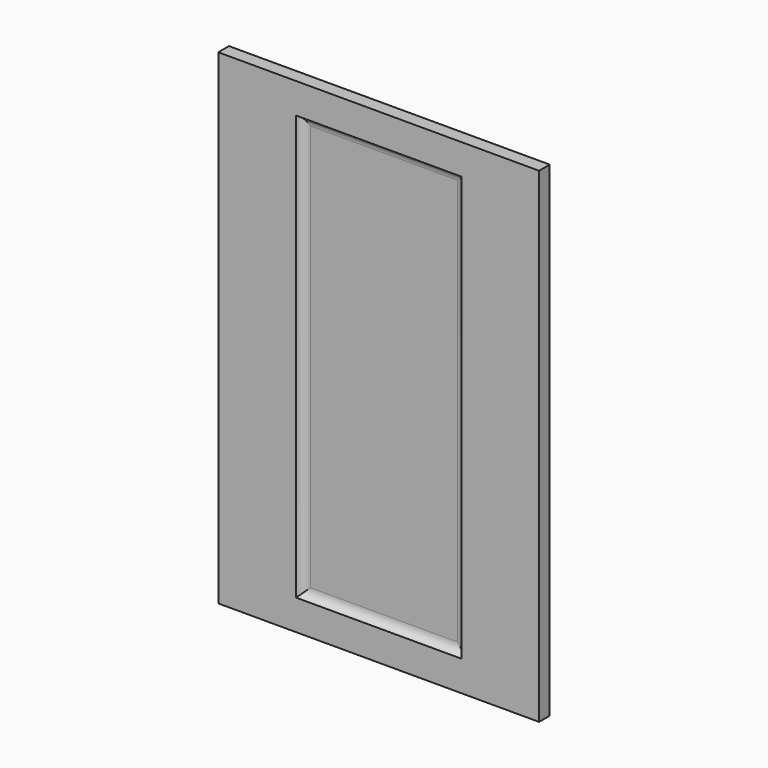
from build123d import *

# Parameters (mm, degrees)
F0_W        = 304.8
F0_H        = 461.01
F1_DEPTH    = 12.7
F2_W        = 157.1649909019
F2_H        = 403.2308459282
F3_DEPTH    = 6.35
F4_T1_DEPTH = 445.8279408996
F4_T3_DEPTH = 199.7620858733


# Not quite as in the source:
# - a fillet or chamfer that OpenCascade refuses, or shapes differently, is made with other operations: its cross-section is extruded or revolved along the edge and cut away or added


with BuildPart() as f1:
    # F0 (on Front) → F1 (new body)
    with BuildSketch(Plane.XZ):
        Rectangle(F0_W, F0_H)
    extrude(amount=F1_DEPTH)

    # F2 (on face) → F3 (cut)
    with BuildSketch(Plane.XZ.offset(12.7)):
        Rectangle(F2_W, F2_H)
    extrude(amount=-F3_DEPTH, mode=Mode.SUBTRACT)

    # F4: fillet of radius 8.89 on 4 edges, made by hand

    # F4_s2 → F4_t1 (join)
    with BuildSketch(Plane.XY.offset(-222.9139704498)):
        with BuildLine():
            ThreePointArc((78.582495451, -12.7), (75.3758676252, -8.1121426782), (70.0630764567, -6.35))
            Line((70.0630764567, -6.35), (78.582495451, -6.35))
            Line((78.582495451, -6.35), (78.582495451, -12.7))
        make_face()
        with BuildLine():
            ThreePointArc((-78.582495451, -12.7), (-75.3758676252, -8.1121426782), (-70.0630764567, -6.35))
            Line((-70.0630764567, -6.35), (-78.582495451, -6.35))
            Line((-78.582495451, -6.35), (-78.582495451, -12.7))
        make_face()
    extrude(amount=F4_T1_DEPTH)

    # F4_s4 → F4_t3 (join)
    with BuildSketch(Plane.YZ.offset(-99.8810429367)):
        with BuildLine():
            ThreePointArc((-12.7, 201.6154229641), (-8.1121426782, 198.4087951383), (-6.35, 193.0960039698))
            Line((-6.35, 193.0960039698), (-6.35, 201.6154229641))
            Line((-6.35, 201.6154229641), (-12.7, 201.6154229641))
        make_face()
        with BuildLine():
            ThreePointArc((-12.7, -201.6154229641), (-8.1121426782, -198.4087951383), (-6.35, -193.0960039698))
            Line((-6.35, -193.0960039698), (-6.35, -201.6154229641))
            Line((-6.35, -201.6154229641), (-12.7, -201.6154229641))
        make_face()
    extrude(amount=F4_T3_DEPTH)


solid = f1.part
